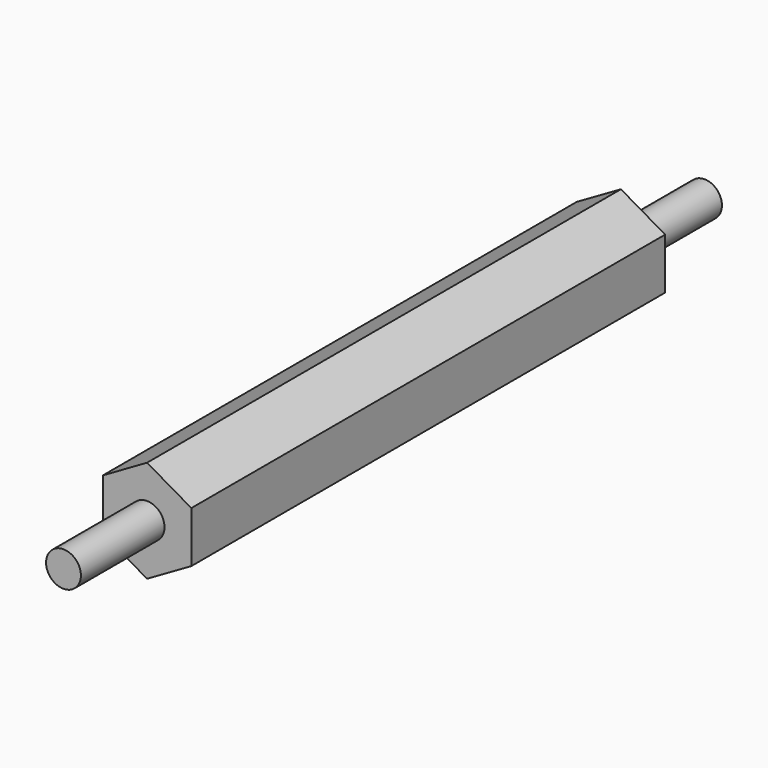
from build123d import *

# Parameters (mm, degrees)
F1_DEPTH = 170
F2_R     = 5
F3_DEPTH = 30
F4_R     = 5
F5_DEPTH = 30


# Not quite as in the source:
# - a feature names something its author has since deleted; it is built from what else it names


with BuildPart() as f1:
    # F0 (on Front) → F1 (new body)
    with BuildSketch(Plane.XZ):
        Polygon((-12.7, 7.3323484187), (-12.7, -7.3323484187), (0, -14.6646968374), (12.7, -7.3323484187), (12.7, 7.3323484187), (0, 14.6646968374), align=None)
    extrude(amount=F1_DEPTH)

    # F2 (on face) → F3 (join)
    with BuildSketch(Plane(origin=(0, 0, 0), x_dir=(-1, 0, 0), z_dir=(0, 1, 0))):
        Circle(F2_R)
    extrude(amount=F3_DEPTH)

    # F4 (on face) → F5 (join)
    with BuildSketch(Plane.XZ.offset(170)):
        Circle(F4_R)
    extrude(amount=F5_DEPTH)


solid = f1.part
